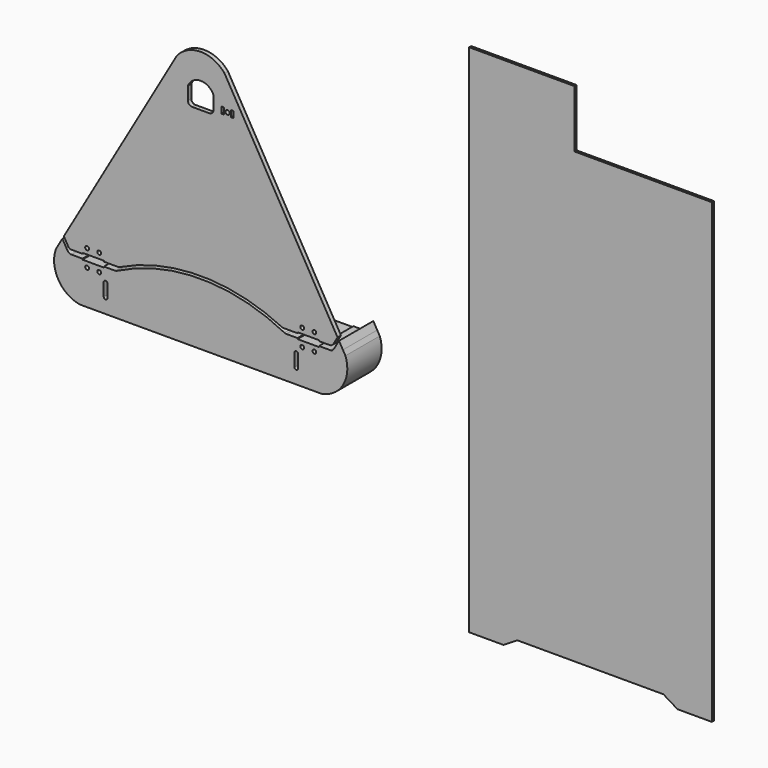
from build123d import *

# Parameters (mm, degrees)
F1_DEPTH = 3
F2_R     = 2.2
F2_W     = 3
F2_H     = 7.5
F2_R_2   = 2.5
F3_DEPTH = 5
F4_DEPTH = 50


# Not quite as in the source:
# - a feature names something its author has since deleted; it is built from what else it names


with BuildPart() as f1:
    # F0 (on Front) → F1 (new body)
    with BuildSketch(Plane.XZ):
        Polygon((-18.5, 233), (-18.5, 300), (-141.2, 300), (-141.2, -300), (-101.2, -300), (-85, -290), (85, -290), (101.5, -300), (141.5, -300), (141.5, 233), align=None)
    extrude(amount=F1_DEPTH)


with BuildPart() as f3:
    # F2 (on Front) → F3 (new body)
    with BuildSketch(Plane.XZ):
        with BuildLine():
            Line((-297.0102405456, -49.3756233624), (-428.6666690787, 178.66))
            ThreePointArc((-428.6666690787, 178.66), (-456.4166690787, 191.66), (-484.1666690787, 178.66))
            Line((-484.1666690787, 178.66), (-615.8230976118, -49.3756233624))
            Line((-615.8230976118, -49.3756233624), (-610.9589453193, -57.8005822687))
            ThreePointArc((-610.9589453193, -57.8005822687), (-609.1288183004, -59.6307092876), (-606.6288183004, -60.3005822687))
            Line((-606.6288183004, -60.3005822687), (-594.219143986, -60.3005822687))
            Line((-594.219143986, -60.3005822687), (-594.219143986, -59.3005822687))
            Line((-594.219143986, -59.3005822687), (-569.219143986, -59.3005822687))
            Line((-569.219143986, -59.3005822687), (-569.219143986, -60.3005822687))
            Line((-569.219143986, -60.3005822687), (-552.9258102304, -60.3005822687))
            ThreePointArc((-552.9258102304, -60.3005822687), (-551.8094969909, -60.1743738883), (-550.7495389858, -59.8021201692))
            ThreePointArc((-550.7495389858, -59.8021201692), (-456.4166690787, -38.1957324085), (-362.0837991717, -59.8021201692))
            ThreePointArc((-362.0837991717, -59.8021201692), (-361.0238411666, -60.1743738883), (-359.9075279271, -60.3005822687))
            Line((-359.9075279271, -60.3005822687), (-343.614543986, -60.3005822687))
            Line((-343.614543986, -60.3005822687), (-343.614543986, -59.3005822687))
            Line((-343.614543986, -59.3005822687), (-318.614543986, -59.3005822687))
            Line((-318.614543986, -59.3005822687), (-318.614543986, -60.3005822687))
            Line((-318.614543986, -60.3005822687), (-306.204519857, -60.3005822687))
            ThreePointArc((-306.204519857, -60.3005822687), (-303.704519857, -59.6307092876), (-301.8743928381, -57.8005822687))
            Line((-301.8743928381, -57.8005822687), (-297.0102405456, -49.3756233624))
        make_face()
        with Locations((-588.769143986, -52.797795045)):
            Circle(F2_R, mode=Mode.SUBTRACT)
        with Locations((-574.669143986, -52.797795045)):
            Circle(F2_R, mode=Mode.SUBTRACT)
        with Locations((-338.164543986, -52.797795045)):
            Circle(F2_R, mode=Mode.SUBTRACT)
        with Locations((-324.064543986, -52.797795045)):
            Circle(F2_R, mode=Mode.SUBTRACT)
        with BuildLine():
            ThreePointArc((-456.8392173046, 161.8821763992), (-456.4166690787, 161.8876722431), (-455.9941208528, 161.8821763992))
            ThreePointArc((-455.9941208528, 161.8821763992), (-447.2262529594, 159.0383885256), (-441.4166690787, 151.8821763992))
            Line((-441.4166690787, 151.8821763992), (-441.4166690787, 136.8821763992))
            ThreePointArc((-441.4166690787, 136.8821763992), (-442.8811351728, 133.3466424933), (-446.4166690787, 131.8821763992))
            Line((-446.4166690787, 131.8821763992), (-466.4166690787, 131.8821763992))
            ThreePointArc((-466.4166690787, 131.8821763992), (-469.9522029846, 133.3466424933), (-471.4166690787, 136.8821763992))
            Line((-471.4166690787, 136.8821763992), (-471.4166690787, 151.8821763992))
            ThreePointArc((-471.4166690787, 151.8821763992), (-465.607085198, 159.0383885256), (-456.8392173046, 161.8821763992))
        make_face(mode=Mode.SUBTRACT)
        with Locations((-430.6666690787, 139.6888568297)):
            Rectangle(F2_W, F2_H, mode=Mode.SUBTRACT)
        with Locations((-425.1666690787, 139.6888568297)):
            Circle(F2_R_2, mode=Mode.SUBTRACT)
        with Locations((-419.6666690787, 139.6888568297)):
            Rectangle(F2_W, F2_H, mode=Mode.SUBTRACT)
    extrude(amount=-F3_DEPTH)


with BuildPart() as f3b:
    # F2 (on Front) → F3, piece 2 (new body)
    with BuildSketch(Plane.XZ):
        with BuildLine():
            Line((-622.1790922267, -60.3845289681), (-625.0157677188, -65.297795045))
            ThreePointArc((-625.0157677188, -65.297795045), (-622.399097968, -95.83), (-597.2657677188, -113.362204955))
            Line((-597.2657677188, -113.362204955), (-578.8804275047, -113.362204955))
            Line((-578.8804275047, -113.362204955), (-315.5675704386, -113.362204955))
            ThreePointArc((-315.5675704386, -113.362204955), (-315.2953712046, -113.314130372), (-315.0235478574, -113.2639740521))
            ThreePointArc((-315.0235478574, -113.2639740521), (-290.2969512012, -95.5900930967), (-287.8175704386, -65.297795045))
            Line((-287.8175704386, -65.297795045), (-290.7543976386, -60.2110611215))
            Line((-290.7543976386, -60.2110611215), (-295.2781897381, -52.3756233624))
            Line((-295.2781897381, -52.3756233624), (-301.2954333646, -62.797795045))
            ThreePointArc((-301.2954333646, -62.797795045), (-303.1255603835, -64.6279220639), (-305.6255603835, -65.297795045))
            Line((-305.6255603835, -65.297795045), (-318.614543986, -65.297795045))
            Line((-318.614543986, -65.297795045), (-318.614543986, -66.356241703))
            Line((-318.614543986, -66.356241703), (-343.614543986, -66.356241703))
            Line((-343.614543986, -66.356241703), (-343.614543986, -65.297795045))
            Line((-343.614543986, -65.297795045), (-356.6028279593, -65.297795045))
            ThreePointArc((-356.6028279593, -65.297795045), (-357.7764477963, -65.1581053723), (-358.8844906049, -64.7468416363))
            ThreePointArc((-358.8844906049, -64.7468416363), (-456.4166690787, -41.1957324085), (-553.9488475525, -64.7468416363))
            ThreePointArc((-553.9488475525, -64.7468416363), (-555.0568903611, -65.1581053723), (-556.2305101981, -65.297795045))
            Line((-556.2305101981, -65.297795045), (-569.219143986, -65.297795045))
            Line((-569.219143986, -65.297795045), (-569.219143986, -66.356241703))
            Line((-569.219143986, -66.356241703), (-594.219143986, -66.356241703))
            Line((-594.219143986, -66.356241703), (-594.219143986, -65.297795045))
            Line((-594.219143986, -65.297795045), (-607.2077777739, -65.297795045))
            ThreePointArc((-607.2077777739, -65.297795045), (-609.7077777739, -64.6279220639), (-611.5379047929, -62.797795045))
            Line((-611.5379047929, -62.797795045), (-613.0562275278, -60.1679829258))
            Line((-613.0562275278, -60.1679829258), (-617.5551484194, -52.3756233624))
            Line((-617.5551484194, -52.3756233624), (-622.1790922267, -60.3845289681))
        make_face()
        with BuildLine():
            ThreePointArc((-569.4157677188, -81.340016621), (-567.2657760294, -79.19), (-565.1157677188, -81.34))
            Line((-565.1157677188, -81.34), (-565.1157677188, -96.34))
            ThreePointArc((-565.1157677188, -96.34), (-567.2769244349, -98.4899710528), (-569.4156519306, -96.3176868683))
            Line((-569.4156519306, -96.3176868683), (-569.4157677188, -81.340016621))
        make_face(mode=Mode.SUBTRACT)
        with Locations((-588.769143986, -72.797795045)):
            Circle(F2_R, mode=Mode.SUBTRACT)
        with Locations((-574.669143986, -72.797795045)):
            Circle(F2_R, mode=Mode.SUBTRACT)
        with BuildLine():
            ThreePointArc((-347.1730506694, -81.293765153), (-345.0004290973, -79.1901243006), (-342.8735478574, -81.34))
            Line((-342.8735478574, -81.34), (-342.8735478574, -96.34))
            ThreePointArc((-342.8735478574, -96.34), (-345.0235833798, -98.4899999997), (-347.1735478562, -96.3399289552))
            Line((-347.1735478562, -96.3399289552), (-347.1730537203, -81.3860927901))
            ThreePointArc((-347.1730537203, -81.3860927901), (-347.1735478562, -81.3399289552), (-347.1730506694, -81.293765153))
        make_face(mode=Mode.SUBTRACT)
        with Locations((-338.164543986, -72.797795045)):
            Circle(F2_R, mode=Mode.SUBTRACT)
        with Locations((-324.064543986, -72.797795045)):
            Circle(F2_R, mode=Mode.SUBTRACT)
    extrude(amount=-F3_DEPTH)


with BuildPart() as f4:
    # F2 (on Front) → F4 (new body)
    with BuildSketch(Plane.XZ):
        with BuildLine():
            Line((-622.1790922267, -60.3845289681), (-625.0157677188, -65.297795045))
            ThreePointArc((-625.0157677188, -65.297795045), (-622.399097968, -95.83), (-597.2657677188, -113.362204955))
            Line((-597.2657677188, -113.362204955), (-578.8804275047, -113.362204955))
            Line((-578.8804275047, -113.362204955), (-315.5675704386, -113.362204955))
            ThreePointArc((-315.5675704386, -113.362204955), (-315.2953712046, -113.314130372), (-315.0235478574, -113.2639740521))
            ThreePointArc((-315.0235478574, -113.2639740521), (-290.2969512012, -95.5900930967), (-287.8175704386, -65.297795045))
            Line((-287.8175704386, -65.297795045), (-290.7543976386, -60.2110611215))
            Line((-290.7543976386, -60.2110611215), (-295.2781897381, -52.3756233624))
            Line((-295.2781897381, -52.3756233624), (-301.2954333646, -62.797795045))
            ThreePointArc((-301.2954333646, -62.797795045), (-303.1255603835, -64.6279220639), (-305.6255603835, -65.297795045))
            Line((-305.6255603835, -65.297795045), (-318.614543986, -65.297795045))
            Line((-318.614543986, -65.297795045), (-318.614543986, -66.356241703))
            Line((-318.614543986, -66.356241703), (-343.614543986, -66.356241703))
            Line((-343.614543986, -66.356241703), (-343.614543986, -65.297795045))
            Line((-343.614543986, -65.297795045), (-356.6028279593, -65.297795045))
            ThreePointArc((-356.6028279593, -65.297795045), (-357.7764477963, -65.1581053723), (-358.8844906049, -64.7468416363))
            ThreePointArc((-358.8844906049, -64.7468416363), (-456.4166690787, -41.1957324085), (-553.9488475525, -64.7468416363))
            ThreePointArc((-553.9488475525, -64.7468416363), (-555.0568903611, -65.1581053723), (-556.2305101981, -65.297795045))
            Line((-556.2305101981, -65.297795045), (-569.219143986, -65.297795045))
            Line((-569.219143986, -65.297795045), (-569.219143986, -66.356241703))
            Line((-569.219143986, -66.356241703), (-594.219143986, -66.356241703))
            Line((-594.219143986, -66.356241703), (-594.219143986, -65.297795045))
            Line((-594.219143986, -65.297795045), (-607.2077777739, -65.297795045))
            ThreePointArc((-607.2077777739, -65.297795045), (-609.7077777739, -64.6279220639), (-611.5379047929, -62.797795045))
            Line((-611.5379047929, -62.797795045), (-613.0562275278, -60.1679829258))
            Line((-613.0562275278, -60.1679829258), (-617.5551484194, -52.3756233624))
            Line((-617.5551484194, -52.3756233624), (-622.1790922267, -60.3845289681))
        make_face()
        with BuildLine():
            ThreePointArc((-569.4157677188, -81.340016621), (-567.2657760294, -79.19), (-565.1157677188, -81.34))
            Line((-565.1157677188, -81.34), (-565.1157677188, -96.34))
            ThreePointArc((-565.1157677188, -96.34), (-567.2769244349, -98.4899710528), (-569.4156519306, -96.3176868683))
            Line((-569.4156519306, -96.3176868683), (-569.4157677188, -81.340016621))
        make_face(mode=Mode.SUBTRACT)
        with Locations((-588.769143986, -72.797795045)):
            Circle(F2_R, mode=Mode.SUBTRACT)
        with Locations((-574.669143986, -72.797795045)):
            Circle(F2_R, mode=Mode.SUBTRACT)
        with BuildLine():
            ThreePointArc((-347.1730506694, -81.293765153), (-345.0004290973, -79.1901243006), (-342.8735478574, -81.34))
            Line((-342.8735478574, -81.34), (-342.8735478574, -96.34))
            ThreePointArc((-342.8735478574, -96.34), (-345.0235833798, -98.4899999997), (-347.1735478562, -96.3399289552))
            Line((-347.1735478562, -96.3399289552), (-347.1730537203, -81.3860927901))
            ThreePointArc((-347.1730537203, -81.3860927901), (-347.1735478562, -81.3399289552), (-347.1730506694, -81.293765153))
        make_face(mode=Mode.SUBTRACT)
        with Locations((-338.164543986, -72.797795045)):
            Circle(F2_R, mode=Mode.SUBTRACT)
        with Locations((-324.064543986, -72.797795045)):
            Circle(F2_R, mode=Mode.SUBTRACT)
    extrude(amount=-F4_DEPTH)


solid = Compound([f1.part, f3.part, f3b.part, f4.part])
